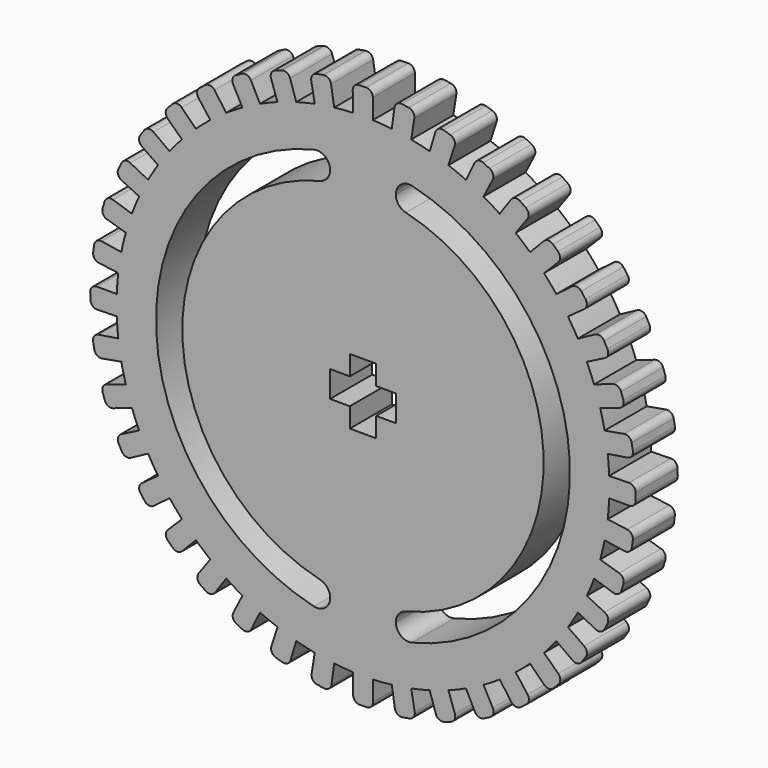
from build123d import *

# Parameters (mm, degrees)
F1_DEPTH = 4
F2_R     = 0.99999
F3_DEPTH = 4


# Not quite as in the source:
# - a fillet or chamfer is up to 0.001 mm smaller than in the source, because OpenCascade refuses the exact size


with BuildPart() as f1:
    # F0 (on Front) → F1 (new body)
    with BuildSketch(Plane.XZ):
        with BuildLine():
            ThreePointArc((-30.5400932527, 19.1737386393), (-30.5288436278, 19.5485886243), (-30.5250932527, 19.9235886243))
            ThreePointArc((-30.5250932527, 19.9235886243), (-30.5288436278, 20.2985886243), (-30.5400932527, 20.6734386092))
            ThreePointArc((-30.5400932527, 20.6734386092), (-30.5828932453, 21.3946966691), (-30.6534498104, 22.1137702394))
            ThreePointArc((-30.6534498104, 22.1137702394), (-30.7559368666, 22.8567348438), (-30.888054573, 23.5950064142))
            ThreePointArc((-30.888054573, 23.5950064142), (-31.0431572453, 24.3006891966), (-31.2253330314, 24.9998722994))
            ThreePointArc((-31.2253330314, 24.9998722994), (-31.4427835722, 25.7176572688), (-31.6887658086, 26.4261717283))
            ThreePointArc((-31.6887658086, 26.4261717283), (-31.9523520182, 27.0989029811), (-32.2416612527, 27.7609794081))
            ThreePointArc((-32.2416612527, 27.7609794081), (-32.5687209242, 28.4359104944), (-32.9225107915, 29.0972218657))
            ThreePointArc((-32.9225107915, 29.0972218657), (-33.2880901711, 29.7204367127), (-33.6774091005, 30.3291039449))
            ThreePointArc((-33.6774091005, 30.3291039449), (-34.1060246082, 30.9445621047), (-34.5589106257, 31.542386707))
            ThreePointArc((-34.5589106257, 31.542386707), (-35.0174813977, 32.1007395304), (-35.497223698, 32.6410101605))
            ThreePointArc((-35.497223698, 32.6410101605), (-36.0168411055, 33.1818407715), (-36.5576717165, 33.701458179))
            ThreePointArc((-36.5576717165, 33.701458179), (-37.0979423466, 34.1812004793), (-37.65629517, 34.6397712513))
            ThreePointArc((-37.65629517, 34.6397712513), (-38.2541197723, 35.0926572688), (-38.8695779321, 35.5212727765))
            ThreePointArc((-38.8695779321, 35.5212727765), (-39.4782451643, 35.9105917059), (-40.1014600113, 36.2761710855))
            ThreePointArc((-40.1014600113, 36.2761710855), (-40.7627713826, 36.6299609528), (-41.4377024689, 36.9570206243))
            ThreePointArc((-41.4377024689, 36.9570206243), (-42.0997788959, 37.2463298588), (-42.7725101487, 37.5099160684))
            ThreePointArc((-42.7725101487, 37.5099160684), (-43.4810246082, 37.7558983048), (-44.1988095776, 37.9733488456))
            ThreePointArc((-44.1988095776, 37.9733488456), (-44.8979926805, 38.1555246317), (-45.6036754628, 38.310627304))
            ThreePointArc((-45.6036754628, 38.310627304), (-46.3419470332, 38.4427450104), (-47.0849116376, 38.5452320666))
            ThreePointArc((-47.0849116376, 38.5452320666), (-47.8039852079, 38.6157886317), (-48.5252432678, 38.6585886243))
            Line((-48.5252432678, 38.6585886243), (-49.2750932527, 38.6735886243))
            Line((-49.2750932527, 38.6735886243), (-50.0249432377, 38.6585886243))
            ThreePointArc((-50.0249432377, 38.6585886243), (-50.7462012976, 38.6157886317), (-51.4652748679, 38.5452320666))
            ThreePointArc((-51.4652748679, 38.5452320666), (-52.2082394723, 38.4427450104), (-52.9465110427, 38.310627304))
            ThreePointArc((-52.9465110427, 38.310627304), (-53.652193825, 38.1555246317), (-54.3513769279, 37.9733488456))
            ThreePointArc((-54.3513769279, 37.9733488456), (-55.0691618973, 37.7558983048), (-55.7776763568, 37.5099160684))
            ThreePointArc((-55.7776763568, 37.5099160684), (-56.4504076096, 37.2463298588), (-57.1124840366, 36.9570206243))
            ThreePointArc((-57.1124840366, 36.9570206243), (-57.7874151229, 36.6299609528), (-58.4487264942, 36.2761710855))
            ThreePointArc((-58.4487264942, 36.2761710855), (-59.0719413412, 35.9105917059), (-59.6806085734, 35.5212727765))
            ThreePointArc((-59.6806085734, 35.5212727765), (-60.2960667332, 35.0926572688), (-60.8938913355, 34.6397712513))
            ThreePointArc((-60.8938913355, 34.6397712513), (-61.4522441589, 34.1812004793), (-61.992514789, 33.701458179))
            ThreePointArc((-61.992514789, 33.701458179), (-62.5333454, 33.1818407715), (-63.0529628075, 32.6410101605))
            ThreePointArc((-63.0529628075, 32.6410101605), (-63.5327051078, 32.1007395304), (-63.9912758798, 31.542386707))
            ThreePointArc((-63.9912758798, 31.542386707), (-64.4441618973, 30.9445621047), (-64.872777405, 30.3291039449))
            ThreePointArc((-64.872777405, 30.3291039449), (-65.2620963344, 29.7204367127), (-65.627675714, 29.0972218657))
            ThreePointArc((-65.627675714, 29.0972218657), (-65.9814655813, 28.4359104944), (-66.3085252528, 27.7609794081))
            ThreePointArc((-66.3085252528, 27.7609794081), (-66.5978344873, 27.0989029811), (-66.8614206969, 26.4261717283))
            ThreePointArc((-66.8614206969, 26.4261717283), (-67.1074029333, 25.7176572688), (-67.3248534741, 24.9998722994))
            ThreePointArc((-67.3248534741, 24.9998722994), (-67.5070292602, 24.3006891966), (-67.6621319325, 23.5950064142))
            ThreePointArc((-67.6621319325, 23.5950064142), (-67.7942496389, 22.8567348438), (-67.8967366951, 22.1137702394))
            ThreePointArc((-67.8967366951, 22.1137702394), (-67.9672932602, 21.3946966691), (-68.0100932527, 20.6734386092))
            ThreePointArc((-68.0100932527, 20.6734386092), (-68.0250932527, 19.9235886243), (-68.0100932527, 19.1737386393))
            ThreePointArc((-68.0100932527, 19.1737386393), (-67.9672932602, 18.4524805794), (-67.8967366951, 17.7334070091))
            ThreePointArc((-67.8967366951, 17.7334070091), (-67.7942496389, 16.9904424047), (-67.6621319325, 16.2521708343))
            ThreePointArc((-67.6621319325, 16.2521708343), (-67.5070292602, 15.546488052), (-67.3248534741, 14.8473049491))
            ThreePointArc((-67.3248534741, 14.8473049491), (-67.1074029333, 14.1295199797), (-66.8614206969, 13.4210055202))
            ThreePointArc((-66.8614206969, 13.4210055202), (-66.5978344873, 12.7482742674), (-66.3085252528, 12.0861978404))
            ThreePointArc((-66.3085252528, 12.0861978404), (-65.9814655813, 11.4112667541), (-65.627675714, 10.7499553828))
            ThreePointArc((-65.627675714, 10.7499553828), (-65.2620963344, 10.1267405358), (-64.872777405, 9.5180733036))
            ThreePointArc((-64.872777405, 9.5180733036), (-64.4441618973, 8.9026151438), (-63.9912758798, 8.3047905415))
            ThreePointArc((-63.9912758798, 8.3047905415), (-63.5327051078, 7.7464377181), (-63.0529628075, 7.206167088))
            ThreePointArc((-63.0529628075, 7.206167088), (-62.5333454, 6.665336477), (-61.992514789, 6.1457190695))
            ThreePointArc((-61.992514789, 6.1457190695), (-61.4522441589, 5.6659767693), (-60.8938913355, 5.2074059973))
            ThreePointArc((-60.8938913355, 5.2074059973), (-60.2960667332, 4.7545199797), (-59.6806085734, 4.325904472))
            ThreePointArc((-59.6806085734, 4.325904472), (-59.0719413412, 3.9365855426), (-58.4487264942, 3.571006163))
            ThreePointArc((-58.4487264942, 3.571006163), (-57.7874151229, 3.2172162957), (-57.1124840366, 2.8901566242))
            ThreePointArc((-57.1124840366, 2.8901566242), (-56.4504076096, 2.6008473897), (-55.7776763568, 2.3372611801))
            ThreePointArc((-55.7776763568, 2.3372611801), (-55.0691618973, 2.0912789437), (-54.3513769279, 1.8738284029))
            ThreePointArc((-54.3513769279, 1.8738284029), (-53.652193825, 1.6916526168), (-52.9465110427, 1.5365499445))
            ThreePointArc((-52.9465110427, 1.5365499445), (-52.2082394723, 1.4044322381), (-51.4652748679, 1.3019451819))
            ThreePointArc((-51.4652748679, 1.3019451819), (-50.7462012976, 1.2313886168), (-50.0249432377, 1.1885886243))
            ThreePointArc((-50.0249432377, 1.1885886243), (-49.2750932528, 1.1735886243), (-48.5252432678, 1.1885886243))
            ThreePointArc((-48.5252432678, 1.1885886243), (-47.8039852079, 1.2313886168), (-47.0849116376, 1.3019451819))
            ThreePointArc((-47.0849116376, 1.3019451819), (-46.3419470332, 1.4044322381), (-45.6036754628, 1.5365499445))
            ThreePointArc((-45.6036754628, 1.5365499445), (-44.8979926805, 1.6916526168), (-44.1988095776, 1.8738284029))
            ThreePointArc((-44.1988095776, 1.8738284029), (-43.4810246082, 2.0912789437), (-42.7725101487, 2.3372611801))
            ThreePointArc((-42.7725101487, 2.3372611801), (-42.0997788959, 2.6008473897), (-41.4377024689, 2.8901566242))
            ThreePointArc((-41.4377024689, 2.8901566242), (-40.7627713826, 3.2172162957), (-40.1014600113, 3.571006163))
            ThreePointArc((-40.1014600113, 3.571006163), (-39.4782451643, 3.9365855426), (-38.8695779321, 4.325904472))
            ThreePointArc((-38.8695779321, 4.325904472), (-38.2541197723, 4.7545199797), (-37.65629517, 5.2074059973))
            ThreePointArc((-37.65629517, 5.2074059973), (-37.0979423466, 5.6659767693), (-36.5576717165, 6.1457190695))
            ThreePointArc((-36.5576717165, 6.1457190695), (-36.0168411055, 6.665336477), (-35.497223698, 7.206167088))
            ThreePointArc((-35.497223698, 7.206167088), (-35.0174813977, 7.7464377181), (-34.5589106257, 8.3047905415))
            ThreePointArc((-34.5589106257, 8.3047905415), (-34.1060246082, 8.9026151438), (-33.6774091005, 9.5180733036))
            ThreePointArc((-33.6774091005, 9.5180733036), (-33.2880901711, 10.1267405358), (-32.9225107915, 10.7499553828))
            ThreePointArc((-32.9225107915, 10.7499553828), (-32.5687209242, 11.4112667541), (-32.2416612527, 12.0861978404))
            ThreePointArc((-32.2416612527, 12.0861978404), (-31.9523520182, 12.7482742674), (-31.6887658086, 13.4210055202))
            ThreePointArc((-31.6887658086, 13.4210055202), (-31.4427835722, 14.1295199797), (-31.2253330314, 14.8473049491))
            ThreePointArc((-31.2253330314, 14.8473049491), (-31.0431572453, 15.546488052), (-30.888054573, 16.2521708343))
            ThreePointArc((-30.888054573, 16.2521708343), (-30.7559368666, 16.9904424047), (-30.6534498104, 17.7334070091))
            ThreePointArc((-30.6534498104, 17.7334070091), (-30.5828932453, 18.4524805794), (-30.5400932527, 19.1737386393))
        make_face()
        with BuildLine():
            Line((-51.7750932527, 35.4739101643), (-51.7750932527, 33.4444059072))
            ThreePointArc((-51.7750932527, 33.4444059072), (-63.0250932527, 19.9235886243), (-51.7750932527, 6.4027713413))
            Line((-51.7750932527, 6.4027713413), (-51.7750932527, 4.3732670842))
            ThreePointArc((-51.7750932527, 4.3732670842), (-65.0250932527, 19.9235886243), (-51.7750932527, 35.4739101643))
        make_face(mode=Mode.SUBTRACT)
        Polygon((-50.2750932527, 20.9235886243), (-50.2750932527, 22.4235886243), (-48.2750932527, 22.4235886243), (-48.2750932527, 20.9235886243), (-46.7750932527, 20.9235886243), (-46.7750932527, 18.9235886243), (-48.2750932527, 18.9235886243), (-48.2750932527, 17.4235886243), (-50.2750932527, 17.4235886243), (-50.2750932527, 18.9235886243), (-51.7750932527, 18.9235886243), (-51.7750932527, 20.9235886243), align=None, mode=Mode.SUBTRACT)
        with BuildLine():
            Line((-46.7750932527, 4.3732670842), (-46.7750932527, 6.4027713413))
            ThreePointArc((-46.7750932527, 6.4027713413), (-35.5250932527, 19.9235886243), (-46.7750932527, 33.4444059072))
            Line((-46.7750932527, 33.4444059072), (-46.7750932527, 35.4739101643))
            ThreePointArc((-46.7750932527, 35.4739101643), (-33.5250932527, 19.9235886243), (-46.7750932527, 4.3732670842))
        make_face(mode=Mode.SUBTRACT)
        with BuildLine():
            Line((-49.2750932527, 38.6735886243), (-48.5252432678, 38.6585886243))
            ThreePointArc((-48.5252432678, 38.6585886243), (-48.9000932527, 38.6698382492), (-49.2750932527, 38.6735886243))
        make_face()
        with BuildLine():
            Line((-50.0249432377, 38.6585886243), (-49.2750932527, 38.6735886243))
            ThreePointArc((-49.2750932527, 38.6735886243), (-49.6500932527, 38.6698382492), (-50.0249432377, 38.6585886243))
        make_face()
    extrude(amount=F1_DEPTH)

    # F2 (radius 1 in the source; OpenCascade refuses exactly that, so slightly less here)
    f2_edges = [f1.edges().sort_by_distance(p)[0] for p in [
        (-51.775093, -2, 35.47391),
        (-51.775093, -2, 33.444406),
        (-51.775093, -2, 4.373267),
        (-51.775093, -2, 6.402771),
        (-46.775093, -2, 6.402771),
        (-46.775093, -2, 4.373267),
        (-46.775093, -2, 35.47391),
        (-46.775093, -2, 33.444406),
    ]]
    fillet(f2_edges, radius=F2_R)

    # F0 (on Front) → F3 (join)
    with BuildSketch(Plane.XZ):
        with BuildLine():
            ThreePointArc((-55.7776763568, 37.5099160684), (-55.0691618973, 37.7558983048), (-54.3513769279, 37.9733488456))
            Line((-54.3513769279, 37.9733488456), (-54.821174874, 39.4192382503))
            ThreePointArc((-54.821174874, 39.4192382503), (-55.0741744889, 39.7124808033), (-55.4606912897, 39.7370727262))
            Line((-55.4606912897, 39.7370727262), (-55.961286014, 39.5632761182))
            ThreePointArc((-55.961286014, 39.5632761182), (-56.247251914, 39.3089729262), (-56.2696408295, 38.9269449876))
            Line((-56.2696408295, 38.9269449876), (-55.7776763568, 37.5099160684))
        make_face()
        with BuildLine():
            ThreePointArc((-52.9465110427, 38.310627304), (-52.2082394723, 38.4427450104), (-51.4652748679, 38.5452320666))
            Line((-51.4652748679, 38.5452320666), (-51.7031018862, 40.0468127637))
            ThreePointArc((-51.7031018862, 40.0468127637), (-51.9071134141, 40.3760228737), (-52.2850245274, 40.4607765781))
            Line((-52.2850245274, 40.4607765781), (-52.8066438794, 40.3674299627))
            ThreePointArc((-52.8066438794, 40.3674299627), (-53.1288708484, 40.1609925876), (-53.2107464554, 39.7871704448))
            Line((-53.2107464554, 39.7871704448), (-52.9465110427, 38.310627304))
        make_face()
        with BuildLine():
            ThreePointArc((-49.2750932527, 38.6735886243), (-48.9000932527, 38.6698382492), (-48.5252432678, 38.6585886243))
            Line((-48.5252432678, 38.6585886243), (-48.5252432678, 40.1788867137))
            ThreePointArc((-48.5252432678, 40.1788867137), (-48.6752432678, 40.5359581351), (-49.0352432678, 40.6787867037))
            Line((-49.0352432678, 40.6787867037), (-49.5650432477, 40.6681885842))
            ThreePointArc((-49.5650432477, 40.6681885842), (-49.9155969884, 40.5147001993), (-50.0549432377, 40.1582885942))
            Line((-50.0549432377, 40.1582885942), (-50.0249432377, 38.6585886243))
            ThreePointArc((-50.0249432377, 38.6585886243), (-49.6500932527, 38.6698382492), (-49.2750932527, 38.6735886243))
        make_face()
        with BuildLine():
            ThreePointArc((-47.0849116376, 38.5452320666), (-46.3419470332, 38.4427450104), (-45.6036754628, 38.310627304))
            Line((-45.6036754628, 38.310627304), (-45.3658484445, 39.8122080012))
            ThreePointArc((-45.3658484445, 39.8122080012), (-45.4581434188, 40.1883484507), (-45.7913679107, 40.38573497))
            Line((-45.7913679107, 40.38573497), (-46.316303085, 40.4581463074))
            ThreePointArc((-46.316303085, 40.4581463074), (-46.6865518007, 40.361386306), (-46.8799375253, 40.0311612753))
            Line((-46.8799375253, 40.0311612753), (-47.0849116376, 38.5452320666))
        make_face()
        with BuildLine():
            ThreePointArc((-44.1988095776, 37.9733488456), (-43.4810246082, 37.7558983048), (-42.7725101487, 37.5099160684))
            Line((-42.7725101487, 37.5099160684), (-42.3027122025, 38.9558054731))
            ThreePointArc((-42.3027122025, 38.9558054731), (-42.3350295425, 39.3417531244), (-42.6332734334, 39.5888372832))
            Line((-42.6332734334, 39.5888372832), (-43.1404181557, 39.7424750701))
            ThreePointArc((-43.1404181557, 39.7424750701), (-43.5212450945, 39.7048260047), (-43.7639084959, 39.4089187844))
            Line((-43.7639084959, 39.4089187844), (-44.1988095776, 37.9733488456))
        make_face()
        with BuildLine():
            ThreePointArc((-41.4377024689, 36.9570206243), (-40.7627713826, 36.6299609528), (-40.1014600113, 36.2761710855))
            Line((-40.1014600113, 36.2761710855), (-39.411259122, 37.6307666019))
            ThreePointArc((-39.411259122, 37.6307666019), (-39.3828030675, 38.017018143), (-39.638722603, 38.3077159093))
            Line((-39.638722603, 38.3077159093), (-40.1155892872, 38.5387970734))
            ThreePointArc((-40.1155892872, 38.5387970734), (-40.4976172258, 38.5611859889), (-40.7835831258, 38.3068827969))
            Line((-40.7835831258, 38.3068827969), (-41.4377024689, 36.9570206243))
        make_face()
        with BuildLine():
            ThreePointArc((-38.8695779321, 35.5212727765), (-38.2541197723, 35.0926572688), (-37.65629517, 34.6397712513))
            Line((-37.65629517, 34.6397712513), (-36.7626863739, 35.8697182421))
            ThreePointArc((-36.7626863739, 35.8697182421), (-36.6741576075, 36.2467628781), (-36.8814511993, 36.5739163082))
            Line((-36.8814511993, 36.5739163082), (-37.316297805, 36.8767508644))
            ThreePointArc((-37.316297805, 36.8767508644), (-37.6901199477, 36.9586264714), (-38.0123469168, 36.7521890962))
            Line((-38.0123469168, 36.7521890962), (-38.8695779321, 35.5212727765))
        make_face()
        with BuildLine():
            ThreePointArc((-36.5576717165, 33.701458179), (-36.0168411055, 33.1818407715), (-35.497223698, 32.6410101605))
            Line((-35.497223698, 32.6410101605), (-34.4222106095, 33.716023249))
            ThreePointArc((-34.4222106095, 33.716023249), (-34.2757890032, 34.0745768896), (-34.4293523951, 34.4301303802))
            Line((-34.4293523951, 34.4301303802), (-34.8114715557, 34.7972615366))
            ThreePointArc((-34.8114715557, 34.7972615366), (-35.1678831607, 34.936607786), (-35.5184369014, 34.783119401))
            Line((-35.5184369014, 34.783119401), (-36.5576717165, 33.701458179))
        make_face()
        with BuildLine():
            ThreePointArc((-34.5589106257, 31.542386707), (-34.1060246082, 30.9445621047), (-33.6774091005, 30.3291039449))
            Line((-33.6774091005, 30.3291039449), (-32.4474621097, 31.2227127409))
            ThreePointArc((-32.4474621097, 31.2227127409), (-32.2467530494, 31.5539466056), (-32.3428050009, 31.9291452498))
            Line((-32.3428050009, 31.9291452498), (-32.6627876746, 32.3515330189))
            ThreePointArc((-32.6627876746, 32.3515330189), (-32.9930127053, 32.5449187435), (-33.3632614211, 32.4481587421))
            Line((-33.3632614211, 32.4481587421), (-34.5589106257, 31.542386707))
        make_face()
        with BuildLine():
            ThreePointArc((-32.9225107915, 29.0972218657), (-32.5687209242, 28.4359104944), (-32.2416612527, 27.7609794081))
            Line((-32.2416612527, 27.7609794081), (-30.8870657363, 28.4511802975))
            ThreePointArc((-30.8870657363, 28.4511802975), (-30.6370113451, 28.7469383091), (-30.6731867386, 29.1325434711))
            Line((-30.6731867386, 29.1325434711), (-30.9231538898, 29.5997872642))
            ThreePointArc((-30.9231538898, 29.5997872642), (-31.2190611101, 29.8424506656), (-31.5998880489, 29.8048016002))
            Line((-31.5998880489, 29.8048016002), (-32.9225107915, 29.0972218657))
        make_face()
        with BuildLine():
            ThreePointArc((-31.6887658086, 26.4261717283), (-31.4427835722, 25.7176572688), (-31.2253330314, 24.9998722994))
            Line((-31.2253330314, 24.9998722994), (-29.7794436267, 25.4696702455))
            ThreePointArc((-29.7794436267, 25.4696702455), (-29.4862010737, 25.7226698604), (-29.4616091508, 26.1091866612))
            Line((-29.4616091508, 26.1091866612), (-29.6354057588, 26.6097813855))
            ThreePointArc((-29.6354057588, 26.6097813855), (-29.8897089508, 26.8957472855), (-30.2717368894, 26.918136201))
            Line((-30.2717368894, 26.918136201), (-31.6887658086, 26.4261717283))
        make_face()
        with BuildLine():
            ThreePointArc((-30.888054573, 23.5950064142), (-30.7559368666, 22.8567348438), (-30.6534498104, 22.1137702394))
            Line((-30.6534498104, 22.1137702394), (-29.1518691133, 22.3515972577))
            ThreePointArc((-29.1518691133, 22.3515972577), (-28.8226590033, 22.5556087856), (-28.7379052989, 22.9335198989))
            Line((-28.7379052989, 22.9335198989), (-28.8312519143, 23.4551392509))
            ThreePointArc((-28.8312519143, 23.4551392509), (-29.0376892894, 23.7773662199), (-29.4115114322, 23.8592418269))
            Line((-29.4115114322, 23.8592418269), (-30.888054573, 23.5950064142))
        make_face()
        with BuildLine():
            ThreePointArc((-30.5400932527, 20.6734386092), (-30.5288436278, 20.2985886243), (-30.5250932527, 19.9235886243))
            ThreePointArc((-30.5250932527, 19.9235886243), (-30.5288436278, 19.5485886243), (-30.5400932527, 19.1737386393))
            Line((-30.5400932527, 19.1737386393), (-29.0197951633, 19.1737386393))
            ThreePointArc((-29.0197951633, 19.1737386393), (-28.6627237419, 19.3237386393), (-28.5198951733, 19.6837386393))
            Line((-28.5198951733, 19.6837386393), (-28.5304932928, 20.2135386193))
            ThreePointArc((-28.5304932928, 20.2135386193), (-28.6839816777, 20.5640923599), (-29.0403932828, 20.7034386092))
            Line((-29.0403932828, 20.7034386092), (-30.5400932527, 20.6734386092))
        make_face()
        with BuildLine():
            ThreePointArc((-58.4487264942, 36.2761710855), (-57.7874151229, 36.6299609528), (-57.1124840366, 36.9570206243))
            Line((-57.1124840366, 36.9570206243), (-57.8026849259, 38.3116161407))
            ThreePointArc((-57.8026849259, 38.3116161407), (-58.0984429376, 38.5616705319), (-58.4840480996, 38.5254951384))
            Line((-58.4840480996, 38.5254951384), (-58.9512918927, 38.2755279872))
            ThreePointArc((-58.9512918927, 38.2755279872), (-59.1939552941, 37.9796207669), (-59.1563062287, 37.5987938281))
            Line((-59.1563062287, 37.5987938281), (-58.4487264942, 36.2761710855))
        make_face()
        with BuildLine():
            ThreePointArc((-60.8938913355, 34.6397712513), (-60.2960667332, 35.0926572688), (-59.6806085734, 35.5212727765))
            Line((-59.6806085734, 35.5212727765), (-60.5742173694, 36.7512197673))
            ThreePointArc((-60.5742173694, 36.7512197673), (-60.9054512341, 36.9519288276), (-61.2806498783, 36.8558768761))
            Line((-61.2806498783, 36.8558768761), (-61.7030376474, 36.5358942024))
            ThreePointArc((-61.7030376474, 36.5358942024), (-61.896423372, 36.2056691717), (-61.7996633706, 35.8354204559))
            Line((-61.7996633706, 35.8354204559), (-60.8938913355, 34.6397712513))
        make_face()
        with BuildLine():
            ThreePointArc((-63.0529628075, 32.6410101605), (-62.5333454, 33.1818407715), (-61.992514789, 33.701458179))
            Line((-61.992514789, 33.701458179), (-63.0675278775, 34.7764712675))
            ThreePointArc((-63.0675278775, 34.7764712675), (-63.4260815181, 34.9228928738), (-63.7816350087, 34.7693294819))
            Line((-63.7816350087, 34.7693294819), (-64.1487661651, 34.3872103213))
            ThreePointArc((-64.1487661651, 34.3872103213), (-64.2881124145, 34.0307987163), (-64.1346240295, 33.6802449756))
            Line((-64.1346240295, 33.6802449756), (-63.0529628075, 32.6410101605))
        make_face()
        with BuildLine():
            ThreePointArc((-64.872777405, 30.3291039449), (-64.4441618973, 30.9445621047), (-63.9912758798, 31.542386707))
            Line((-63.9912758798, 31.542386707), (-65.2212228706, 32.4359955031))
            ThreePointArc((-65.2212228706, 32.4359955031), (-65.5982675066, 32.5245242695), (-65.9254209367, 32.3172306777))
            Line((-65.9254209367, 32.3172306777), (-66.2282554929, 31.882384072))
            ThreePointArc((-66.2282554929, 31.882384072), (-66.3101310999, 31.5085619293), (-66.1036937247, 31.1863349603))
            Line((-66.1036937247, 31.1863349603), (-64.872777405, 30.3291039449))
        make_face()
        with BuildLine():
            ThreePointArc((-66.3085252528, 27.7609794081), (-65.9814655813, 28.4359104944), (-65.627675714, 29.0972218657))
            Line((-65.627675714, 29.0972218657), (-66.9822712304, 29.787422755))
            ThreePointArc((-66.9822712304, 29.787422755), (-67.3685227714, 29.8158788095), (-67.6592205378, 29.559959274))
            Line((-67.6592205378, 29.559959274), (-67.8903017019, 29.0830925898))
            ThreePointArc((-67.8903017019, 29.0830925898), (-67.9126906174, 28.7010646512), (-67.6583874254, 28.4150987512))
            Line((-67.6583874254, 28.4150987512), (-66.3085252528, 27.7609794081))
        make_face()
        with BuildLine():
            ThreePointArc((-67.3248534741, 24.9998722994), (-67.1074029333, 25.7176572688), (-66.8614206969, 26.4261717283))
            Line((-66.8614206969, 26.4261717283), (-68.3073101016, 26.8959696745))
            ThreePointArc((-68.3073101016, 26.8959696745), (-68.6932577529, 26.8636523345), (-68.9403419117, 26.5654084436))
            Line((-68.9403419117, 26.5654084436), (-69.0939796986, 26.0582637213))
            ThreePointArc((-69.0939796986, 26.0582637213), (-69.0563306332, 25.6774367825), (-68.7604234129, 25.4347733811))
            Line((-68.7604234129, 25.4347733811), (-67.3248534741, 24.9998722994))
        make_face()
        with BuildLine():
            ThreePointArc((-67.8967366951, 22.1137702394), (-67.7942496389, 22.8567348438), (-67.6621319325, 23.5950064142))
            Line((-67.6621319325, 23.5950064142), (-69.1637126297, 23.8328334325))
            ThreePointArc((-69.1637126297, 23.8328334325), (-69.5398530792, 23.7405384582), (-69.7372395985, 23.4073139663))
            Line((-69.7372395985, 23.4073139663), (-69.8096509359, 22.8823787921))
            ThreePointArc((-69.8096509359, 22.8823787921), (-69.7128909345, 22.5121300763), (-69.3826659038, 22.3187443517))
            Line((-69.3826659038, 22.3187443517), (-67.8967366951, 22.1137702394))
        make_face()
        with BuildLine():
            Line((-69.1386750733, 15.9879354216), (-67.6621319325, 16.2521708343))
            ThreePointArc((-67.6621319325, 16.2521708343), (-67.7942496389, 16.9904424047), (-67.8967366951, 17.7334070091))
            Line((-67.8967366951, 17.7334070091), (-69.3983173922, 17.4955799908))
            ThreePointArc((-69.3983173922, 17.4955799908), (-69.7275275022, 17.2915684629), (-69.8122812066, 16.9136573496))
            Line((-69.8122812066, 16.9136573496), (-69.7189345912, 16.3920379976))
            ThreePointArc((-69.7189345912, 16.3920379976), (-69.5124972161, 16.0698110286), (-69.1386750733, 15.9879354216))
        make_face()
        with BuildLine():
            Line((-68.2784496161, 12.9290410475), (-66.8614206969, 13.4210055202))
            ThreePointArc((-66.8614206969, 13.4210055202), (-67.1074029333, 14.1295199797), (-67.3248534741, 14.8473049491))
            Line((-67.3248534741, 14.8473049491), (-68.7707428788, 14.377507003))
            ThreePointArc((-68.7707428788, 14.377507003), (-69.0639854318, 14.1245073881), (-69.0885773547, 13.7379905873))
            Line((-69.0885773547, 13.7379905873), (-68.9147807467, 13.237395863))
            ThreePointArc((-68.9147807467, 13.237395863), (-68.6604775547, 12.951429963), (-68.2784496161, 12.9290410475))
        make_face()
        with BuildLine():
            Line((-66.9502984566, 10.0423756483), (-65.627675714, 10.7499553828))
            ThreePointArc((-65.627675714, 10.7499553828), (-65.9814655813, 11.4112667541), (-66.3085252528, 12.0861978404))
            Line((-66.3085252528, 12.0861978404), (-67.6631207692, 11.3959969511))
            ThreePointArc((-67.6631207692, 11.3959969511), (-67.9131751604, 11.1002389394), (-67.8769997669, 10.7146337774))
            Line((-67.8769997669, 10.7146337774), (-67.6270326157, 10.2473899843))
            ThreePointArc((-67.6270326157, 10.2473899843), (-67.3311253954, 10.0047265829), (-66.9502984566, 10.0423756483))
        make_face()
        with BuildLine():
            Line((-69.5097932227, 19.1437386393), (-68.0100932527, 19.1737386393))
            ThreePointArc((-68.0100932527, 19.1737386393), (-68.0250932527, 19.9235886243), (-68.0100932527, 20.6734386092))
            Line((-68.0100932527, 20.6734386092), (-69.5303913422, 20.6734386092))
            ThreePointArc((-69.5303913422, 20.6734386092), (-69.8874627636, 20.5234386092), (-70.0302913322, 20.1634386092))
            Line((-70.0302913322, 20.1634386092), (-70.0196932127, 19.6336386293))
            ThreePointArc((-70.0196932127, 19.6336386293), (-69.8662048278, 19.2830848886), (-69.5097932227, 19.1437386393))
        make_face()
        with BuildLine():
            Line((-65.1869250844, 7.3990185064), (-63.9912758798, 8.3047905415))
            ThreePointArc((-63.9912758798, 8.3047905415), (-64.4441618973, 8.9026151438), (-64.872777405, 9.5180733036))
            Line((-64.872777405, 9.5180733036), (-66.1027243958, 8.6244645076))
            ThreePointArc((-66.1027243958, 8.6244645076), (-66.3034334561, 8.2932306429), (-66.2073815046, 7.9180319987))
            Line((-66.2073815046, 7.9180319987), (-65.8873988309, 7.4956442296))
            ThreePointArc((-65.8873988309, 7.4956442296), (-65.5571738002, 7.302258505), (-65.1869250844, 7.3990185064))
        make_face()
        with BuildLine():
            Line((-63.0317496041, 5.0640578475), (-61.992514789, 6.1457190695))
            ThreePointArc((-61.992514789, 6.1457190695), (-62.5333454, 6.665336477), (-63.0529628075, 7.206167088))
            Line((-63.0529628075, 7.206167088), (-64.127975896, 6.1311539995))
            ThreePointArc((-64.127975896, 6.1311539995), (-64.2743975023, 5.7726003589), (-64.1208341104, 5.4170468683))
            Line((-64.1208341104, 5.4170468683), (-63.7387149498, 5.0499157119))
            ThreePointArc((-63.7387149498, 5.0499157119), (-63.3823033448, 4.9105694625), (-63.0317496041, 5.0640578475))
        make_face()
        with BuildLine():
            Line((-60.5378395887, 3.0949881523), (-59.6806085734, 4.325904472))
            ThreePointArc((-59.6806085734, 4.325904472), (-60.2960667332, 4.7545199797), (-60.8938913355, 5.2074059973))
            Line((-60.8938913355, 5.2074059973), (-61.7875001316, 3.9774590064))
            ThreePointArc((-61.7875001316, 3.9774590064), (-61.876028898, 3.6004143704), (-61.6687353062, 3.2732609403))
            Line((-61.6687353062, 3.2732609403), (-61.2338887005, 2.9704263841))
            ThreePointArc((-61.2338887005, 2.9704263841), (-60.8600665578, 2.8885507771), (-60.5378395887, 3.0949881523))
        make_face()
        with BuildLine():
            Line((-57.7666033797, 1.5402944516), (-57.1124840366, 2.8901566242))
            ThreePointArc((-57.1124840366, 2.8901566242), (-57.7874151229, 3.2172162957), (-58.4487264942, 3.571006163))
            Line((-58.4487264942, 3.571006163), (-59.1389273835, 2.2164106466))
            ThreePointArc((-59.1389273835, 2.2164106466), (-59.167383438, 1.8301591056), (-58.9114639025, 1.5394613392))
            Line((-58.9114639025, 1.5394613392), (-58.4345972183, 1.3083801751))
            ThreePointArc((-58.4345972183, 1.3083801751), (-58.0525692797, 1.2859912596), (-57.7666033797, 1.5402944516))
        make_face()
        with BuildLine():
            Line((-54.7862780096, 0.4382584641), (-54.3513769279, 1.8738284029))
            ThreePointArc((-54.3513769279, 1.8738284029), (-55.0691618973, 2.0912789437), (-55.7776763568, 2.3372611801))
            Line((-55.7776763568, 2.3372611801), (-56.247474303, 0.8913717754))
            ThreePointArc((-56.247474303, 0.8913717754), (-56.215156963, 0.5054241241), (-55.9169130721, 0.2583399653))
            Line((-55.9169130721, 0.2583399653), (-55.4097683498, 0.1047021784))
            ThreePointArc((-55.4097683498, 0.1047021784), (-55.028941411, 0.1423512438), (-54.7862780096, 0.4382584641))
        make_face()
        with BuildLine():
            Line((-51.6702489802, -0.1839840268), (-51.4652748679, 1.3019451819))
            ThreePointArc((-51.4652748679, 1.3019451819), (-52.2082394723, 1.4044322381), (-52.9465110427, 1.5365499445))
            Line((-52.9465110427, 1.5365499445), (-53.184338061, 0.0349692473))
            ThreePointArc((-53.184338061, 0.0349692473), (-53.0920430867, -0.3411712022), (-52.7588185948, -0.5385577214))
            Line((-52.7588185948, -0.5385577214), (-52.2338834205, -0.6109690589))
            ThreePointArc((-52.2338834205, -0.6109690589), (-51.8636347048, -0.5142090575), (-51.6702489802, -0.1839840268))
        make_face()
        with BuildLine():
            Line((-48.4952432678, -0.3111113457), (-48.5252432678, 1.1885886243))
            ThreePointArc((-48.5252432678, 1.1885886243), (-49.2750932528, 1.1735886243), (-50.0249432377, 1.1885886243))
            Line((-50.0249432377, 1.1885886243), (-50.0249432377, -0.3317094652))
            ThreePointArc((-50.0249432377, -0.3317094652), (-49.8749432377, -0.6887808866), (-49.5149432377, -0.8316094552))
            Line((-49.5149432377, -0.8316094552), (-48.9851432578, -0.8210113357))
            ThreePointArc((-48.9851432578, -0.8210113357), (-48.6345895171, -0.6675229508), (-48.4952432678, -0.3111113457))
        make_face()
        with BuildLine():
            Line((-45.3394400501, 0.0600068037), (-45.6036754628, 1.5365499445))
            ThreePointArc((-45.6036754628, 1.5365499445), (-46.3419470332, 1.4044322381), (-47.0849116376, 1.3019451819))
            Line((-47.0849116376, 1.3019451819), (-46.8470846193, -0.1996355152))
            ThreePointArc((-46.8470846193, -0.1996355152), (-46.6430730914, -0.5288456252), (-46.2651619781, -0.6135993296))
            Line((-46.2651619781, -0.6135993296), (-45.7435426261, -0.5202527142))
            ThreePointArc((-45.7435426261, -0.5202527142), (-45.4213156571, -0.3138153391), (-45.3394400501, 0.0600068037))
        make_face()
        with BuildLine():
            Line((-42.280545676, 0.9202322609), (-42.7725101487, 2.3372611801))
            ThreePointArc((-42.7725101487, 2.3372611801), (-43.4810246082, 2.0912789437), (-44.1988095776, 1.8738284029))
            Line((-44.1988095776, 1.8738284029), (-43.7290116315, 0.4279389982))
            ThreePointArc((-43.7290116315, 0.4279389982), (-43.4760120166, 0.1346964452), (-43.0894952158, 0.1101045224))
            Line((-43.0894952158, 0.1101045224), (-42.5889004915, 0.2839011303))
            ThreePointArc((-42.5889004915, 0.2839011303), (-42.3029345915, 0.5382043223), (-42.280545676, 0.9202322609))
        make_face()
        with BuildLine():
            Line((-39.3938802768, 2.2483834204), (-40.1014600113, 3.571006163))
            ThreePointArc((-40.1014600113, 3.571006163), (-40.7627713826, 3.2172162957), (-41.4377024689, 2.8901566242))
            Line((-41.4377024689, 2.8901566242), (-40.7475015796, 1.5355611078))
            ThreePointArc((-40.7475015796, 1.5355611078), (-40.4517435679, 1.2855067166), (-40.0661384059, 1.3216821101))
            Line((-40.0661384059, 1.3216821101), (-39.5988946128, 1.5716492614))
            ThreePointArc((-39.5988946128, 1.5716492614), (-39.3562312114, 1.8675564816), (-39.3938802768, 2.2483834204))
        make_face()
        with BuildLine():
            Line((-36.7505231349, 4.0117567926), (-37.65629517, 5.2074059973))
            ThreePointArc((-37.65629517, 5.2074059973), (-38.2541197723, 4.7545199797), (-38.8695779321, 4.325904472))
            Line((-38.8695779321, 4.325904472), (-37.9759691361, 3.0959574812))
            ThreePointArc((-37.9759691361, 3.0959574812), (-37.6447352714, 2.8952484209), (-37.2695366272, 2.9913003724))
            Line((-37.2695366272, 2.9913003724), (-36.8471488581, 3.3112830461))
            ThreePointArc((-36.8471488581, 3.3112830461), (-36.6537631335, 3.6415080768), (-36.7505231349, 4.0117567926))
        make_face()
        with BuildLine():
            Line((-34.415562476, 6.1669322729), (-35.497223698, 7.206167088))
            ThreePointArc((-35.497223698, 7.206167088), (-36.0168411055, 6.665336477), (-36.5576717165, 6.1457190695))
            Line((-36.5576717165, 6.1457190695), (-35.482658628, 5.070705981))
            ThreePointArc((-35.482658628, 5.070705981), (-35.1241049874, 4.9242843747), (-34.7685514968, 5.0778477666))
            Line((-34.7685514968, 5.0778477666), (-34.4014203404, 5.4599669272))
            ThreePointArc((-34.4014203404, 5.4599669272), (-34.262074091, 5.8163785322), (-34.415562476, 6.1669322729))
        make_face()
        with BuildLine():
            Line((-32.4464927808, 8.6608422883), (-33.6774091005, 9.5180733036))
            ThreePointArc((-33.6774091005, 9.5180733036), (-34.1060246082, 8.9026151438), (-34.5589106257, 8.3047905415))
            Line((-34.5589106257, 8.3047905415), (-33.3289636349, 7.4111817454))
            ThreePointArc((-33.3289636349, 7.4111817454), (-32.9519189989, 7.322652979), (-32.6247655688, 7.5299465708))
            Line((-32.6247655688, 7.5299465708), (-32.3219310126, 7.9647931765))
            ThreePointArc((-32.3219310126, 7.9647931765), (-32.2400554056, 8.3386153192), (-32.4464927808, 8.6608422883))
        make_face()
        with BuildLine():
            Line((-29.7897630926, 14.4124038674), (-31.2253330314, 14.8473049491))
            ThreePointArc((-31.2253330314, 14.8473049491), (-31.4427835722, 14.1295199797), (-31.6887658086, 13.4210055202))
            Line((-31.6887658086, 13.4210055202), (-30.2428764039, 12.951207574))
            ThreePointArc((-30.2428764039, 12.951207574), (-29.8569287526, 12.983524914), (-29.6098445938, 13.2817688049))
            Line((-29.6098445938, 13.2817688049), (-29.4562068069, 13.7889135272))
            ThreePointArc((-29.4562068069, 13.7889135272), (-29.4938558723, 14.169740466), (-29.7897630926, 14.4124038674))
        make_face()
        with BuildLine():
            Line((-29.1675206017, 17.5284328968), (-30.6534498104, 17.7334070091))
            ThreePointArc((-30.6534498104, 17.7334070091), (-30.7559368666, 16.9904424047), (-30.888054573, 16.2521708343))
            Line((-30.888054573, 16.2521708343), (-29.3864738758, 16.014343816))
            ThreePointArc((-29.3864738758, 16.014343816), (-29.0103334263, 16.1066387903), (-28.812946907, 16.4398632822))
            Line((-28.812946907, 16.4398632822), (-28.7405355696, 16.9647984565))
            ThreePointArc((-28.7405355696, 16.9647984565), (-28.837295571, 17.3350471722), (-29.1675206017, 17.5284328968))
        make_face()
        with BuildLine():
            Line((-30.8917990801, 11.4320784973), (-32.2416612527, 12.0861978404))
            ThreePointArc((-32.2416612527, 12.0861978404), (-32.5687209242, 11.4112667541), (-32.9225107915, 10.7499553828))
            Line((-32.9225107915, 10.7499553828), (-31.5679152751, 10.0597544935))
            ThreePointArc((-31.5679152751, 10.0597544935), (-31.1816637341, 10.031298439), (-30.8909659677, 10.2872179745))
            Line((-30.8909659677, 10.2872179745), (-30.6598848036, 10.7640846588))
            ThreePointArc((-30.6598848036, 10.7640846588), (-30.6374958881, 11.1461125973), (-30.8917990801, 11.4320784973))
        make_face()
    extrude(amount=F3_DEPTH)


solid = f1.part
